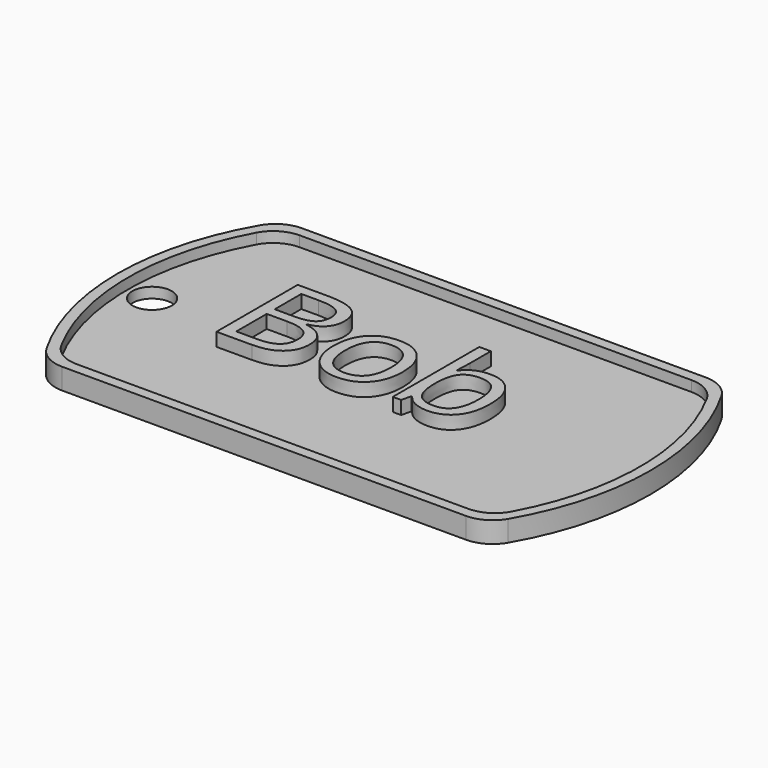
from build123d import *

# Parameters (mm, degrees)
F0_R         = 1.8739594118
F1_DEPTH     = 1
F3_DEPTH     = 1
F4_TEXT_SIZE = 13.5534433884
F5_DEPTH     = 1.27


# Not quite as in the source:
# - Text() gives the source's letters only with a copy of the font that has no kerning and outlines rounded to 1/6400 em; it was checked with that copy


with BuildPart() as f1:
    # F0 (on Top) → F1 (new body)
    with BuildSketch(Plane.XY):
        with BuildLine():
            ThreePointArc((-19.2474145991, 14.2875), (-20.8349145991, 13.862130657), (-21.9970452561, 12.7))
            ThreePointArc((-21.9970452561, 12.7), (-25.4, 0), (-21.9970452561, -12.7))
            ThreePointArc((-21.9970452561, -12.7), (-20.8349145991, -13.862130657), (-19.2474145991, -14.2875))
            Line((-19.2474145991, -14.2875), (19.2474145991, -14.2875))
            ThreePointArc((19.2474145991, -14.2875), (20.8349145991, -13.862130657), (21.9970452561, -12.7))
            ThreePointArc((21.9970452561, -12.7), (25.4, 0), (21.9970452561, 12.7))
            ThreePointArc((21.9970452561, 12.7), (20.8349145991, 13.862130657), (19.2474145991, 14.2875))
            Line((19.2474145991, 14.2875), (-19.2474145991, 14.2875))
        make_face()
        with Locations((-22.0978986472, 0)):
            Circle(F0_R, mode=Mode.SUBTRACT)
    extrude(amount=F1_DEPTH)

    # F2 (on face) → F3 (join)
    with BuildSketch(Plane.XY.offset(1)):
        with BuildLine():
            Line((19.2474145991, 14.2875), (-19.2474145991, 14.2875))
            ThreePointArc((-19.2474145991, 14.2875), (-20.8349145991, 13.862130657), (-21.9970452561, 12.7))
            ThreePointArc((-21.9970452561, 12.7), (-25.4, 0), (-21.9970452561, -12.7))
            ThreePointArc((-21.9970452561, -12.7), (-20.8349145991, -13.862130657), (-19.2474145991, -14.2875))
            Line((-19.2474145991, -14.2875), (19.2474145991, -14.2875))
            ThreePointArc((19.2474145991, -14.2875), (20.8349145991, -13.862130657), (21.9970452561, -12.7))
            ThreePointArc((21.9970452561, -12.7), (25.4, 0), (21.9970452561, 12.7))
            ThreePointArc((21.9970452561, 12.7), (20.8349145991, 13.862130657), (19.2474145991, 14.2875))
        make_face()
        with BuildLine():
            ThreePointArc((-21.4526124879, 11.6252061249), (-20.2856017842, 12.8404540819), (-18.6611352482, 13.2875))
            Line((-18.6611352482, 13.2875), (18.6611352482, 13.2875))
            ThreePointArc((18.6611352482, 13.2875), (20.2856017842, 12.8404540819), (21.4526124879, 11.6252061249))
            ThreePointArc((21.4526124879, 11.6252061249), (24.4, 0), (21.4526124879, -11.6252061249))
            ThreePointArc((21.4526124879, -11.6252061249), (20.2856017842, -12.8404540819), (18.6611352482, -13.2875))
            Line((18.6611352482, -13.2875), (-18.6611352482, -13.2875))
            ThreePointArc((-18.6611352482, -13.2875), (-20.2856017842, -12.8404540819), (-21.4526124879, -11.6252061249))
            ThreePointArc((-21.4526124879, -11.6252061249), (-24.4, 0), (-21.4526124879, 11.6252061249))
        make_face(mode=Mode.SUBTRACT)
    extrude(amount=F3_DEPTH)

    # F4 (on face) → F5 (join)
    with BuildSketch(Plane.XY.offset(1)):
        with Locations((-14.8030400997, -3.1132530072)):
            Text('Bob', F4_TEXT_SIZE, font='Open Sans', text_align=(TextAlign.LEFT, TextAlign.BOTTOM))
    extrude(amount=F5_DEPTH)


solid = f1.part
